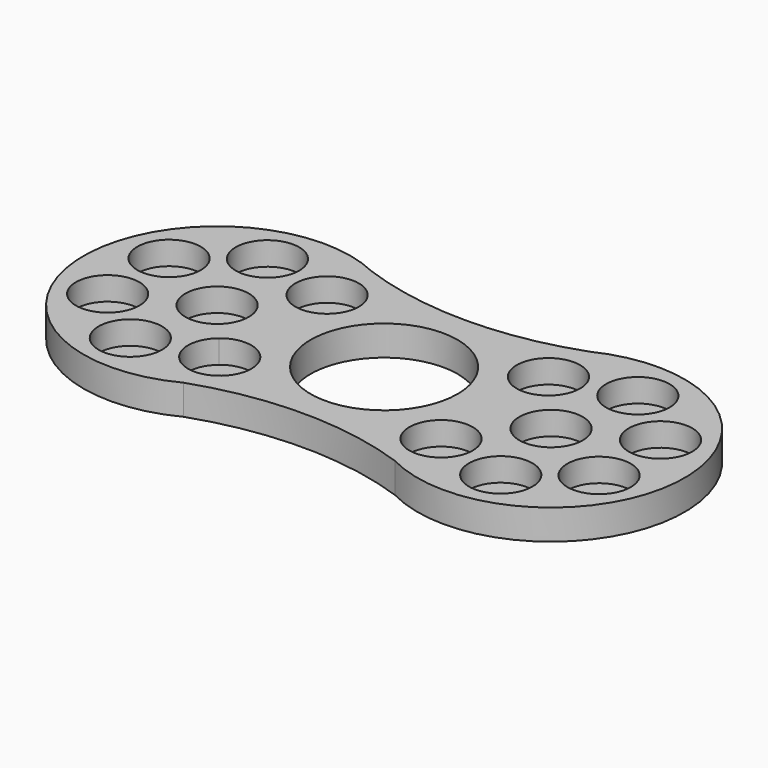
from build123d import *

# Parameters (mm, degrees)
F0_R     = 4.75
F1_DEPTH = 4.5
F2_DEPTH = 1


# Not quite as in the source:
# - a feature names something its author has since deleted; it is built from what else it names


with BuildPart() as f1:
    # F0 (on Top) → F1 (new body)
    with BuildSketch(Plane.XY):
        with BuildLine():
            ThreePointArc((-15.8212677669, -17.7693802535), (0, -15.0870091218), (15.8212677669, -17.7693802535))
            ThreePointArc((15.8212677669, -17.7693802535), (44.9980398453, -0.2800041916), (16.3223672692, 18.019397609))
            ThreePointArc((16.3223672692, 18.019397609), (0, 15.1589625906), (-16.3223672692, 18.019397609))
            ThreePointArc((-16.3223672692, 18.019397609), (-44.9980398453, -0.2800041916), (-15.8212677669, -17.7693802535))
        make_face()
        with Locations((-27.7271234226, -12.8301069662)):
            Circle(F0_R, mode=Mode.SUBTRACT)
        with BuildLine():
            ThreePointArc((-11.8187225704, -10.0480051668), (-18.5761593137, -14.3529671553), (-19.6219637164, -6.409294062))
            ThreePointArc((-19.6219637164, -6.409294062), (-14.5612858272, -5.7430431784), (-11.8187225704, -10.0480051668))
        make_face(mode=Mode.SUBTRACT)
        with Locations((-36.7892470891, -5.75)):
            Circle(F0_R, mode=Mode.SUBTRACT)
        with Locations((16.5687225704, -10.0480051668)):
            Circle(F0_R, mode=Mode.SUBTRACT)
        with Locations((27.7271234226, -12.8301069662)):
            Circle(F0_R, mode=Mode.SUBTRACT)
        with Locations((36.7892470891, -5.75)):
            Circle(F0_R, mode=Mode.SUBTRACT)
        with BuildLine():
            ThreePointArc((-21.946758854, 3.6387111048), (-20.6950380116, 2.0074367433), (-20.25, 0))
            ThreePointArc((-20.25, 0), (-20.6950380116, -2.0074367433), (-21.946758854, -3.6387111048))
            ThreePointArc((-21.946758854, -3.6387111048), (-29.75, 0), (-21.946758854, 3.6387111048))
        make_face(mode=Mode.SUBTRACT)
        with Locations((-36.7892470891, 5.75)):
            Circle(F0_R, mode=Mode.SUBTRACT)
        with Locations((-27.7271234226, 12.8301069662)):
            Circle(F0_R, mode=Mode.SUBTRACT)
        with BuildLine():
            ThreePointArc((-11.8187225704, 10.0480051668), (-14.5612858272, 5.7430431784), (-19.6219637164, 6.409294062))
            ThreePointArc((-19.6219637164, 6.409294062), (-18.5761593137, 14.3529671553), (-11.8187225704, 10.0480051668))
        make_face(mode=Mode.SUBTRACT)
        with BuildLine():
            ThreePointArc((-11, 0), (0, 11), (11, 0))
            ThreePointArc((11, 0), (0, -11), (-11, 0))
        make_face(mode=Mode.SUBTRACT)
        with Locations((25, 0)):
            Circle(F0_R, mode=Mode.SUBTRACT)
        with Locations((36.7892470891, 5.75)):
            Circle(F0_R, mode=Mode.SUBTRACT)
        with Locations((16.5687225704, 10.0480051668)):
            Circle(F0_R, mode=Mode.SUBTRACT)
        with Locations((27.7271234226, 12.8301069662)):
            Circle(F0_R, mode=Mode.SUBTRACT)
    extrude(amount=F1_DEPTH)

    # F0 (on Top) → F2 (join)
    with BuildSketch(Plane.XY):
        with BuildLine():
            Line((-25, 0), (-20.25, 0))
            ThreePointArc((-20.25, 0), (-20.6950380116, 2.0074367433), (-21.946758854, 3.6387111048))
            Line((-21.946758854, 3.6387111048), (-25, 0))
        make_face()
        with BuildLine():
            Line((-25, 0), (-21.946758854, 3.6387111048))
            ThreePointArc((-21.946758854, 3.6387111048), (-29.75, 0), (-21.946758854, -3.6387111048))
            Line((-21.946758854, -3.6387111048), (-25, 0))
        make_face()
        with BuildLine():
            ThreePointArc((-21.946758854, -3.6387111048), (-20.6950380116, -2.0074367433), (-20.25, 0))
            Line((-20.25, 0), (-25, 0))
            Line((-25, 0), (-21.946758854, -3.6387111048))
        make_face()
        with Locations((25, 0)):
            Circle(F0_R)
        with BuildLine():
            ThreePointArc((-11.8187225704, 10.0480051668), (-18.5761593137, 14.3529671553), (-19.6219637164, 6.409294062))
            ThreePointArc((-19.6219637164, 6.409294062), (-14.5612858272, 5.7430431784), (-11.8187225704, 10.0480051668))
        make_face()
        with Locations((-27.7271234226, 12.8301069662)):
            Circle(F0_R)
        with Locations((-36.7892470891, 5.75)):
            Circle(F0_R)
        with Locations((-36.7892470891, -5.75)):
            Circle(F0_R)
        with Locations((-27.7271234226, -12.8301069662)):
            Circle(F0_R)
        with BuildLine():
            ThreePointArc((-11.8187225704, -10.0480051668), (-14.5612858272, -5.7430431784), (-19.6219637164, -6.409294062))
            ThreePointArc((-19.6219637164, -6.409294062), (-18.5761593137, -14.3529671553), (-11.8187225704, -10.0480051668))
        make_face()
        with Locations((16.5687225704, 10.0480051668)):
            Circle(F0_R)
        with Locations((27.7271234226, 12.8301069662)):
            Circle(F0_R)
        with Locations((36.7892470891, 5.75)):
            Circle(F0_R)
        with Locations((36.7892470891, -5.75)):
            Circle(F0_R)
        with Locations((27.7271234226, -12.8301069662)):
            Circle(F0_R)
        with Locations((16.5687225704, -10.0480051668)):
            Circle(F0_R)
    extrude(amount=F2_DEPTH)


solid = f1.part
